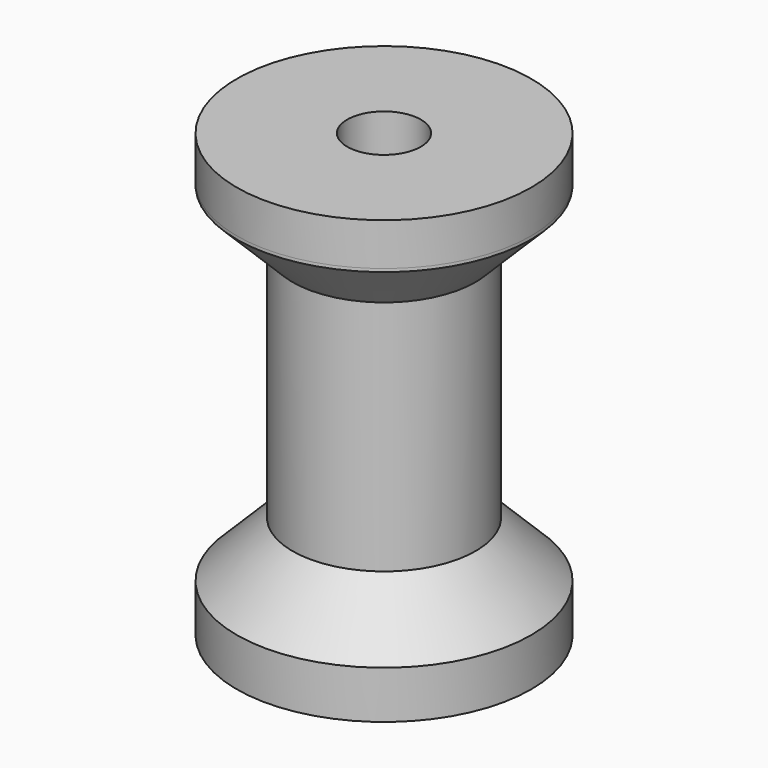
from build123d import *

# Parameters (mm, degrees)
F0_R         = 12.7
F1_DEPTH     = 38.1
F2_W         = 10.2602215484
F2_H         = 30.5833565071
F4_R         = 3.175
F5_DEPTH     = 50.8
F6_S5_R      = 12.7
F6_T6_DEPTH  = 20
F6_S11_R     = 12.7
F6_T12_DEPTH = 20


# Not quite as in the source:
# - a fillet or chamfer that OpenCascade refuses, or shapes differently, is made with other operations: its cross-section is extruded or revolved along the edge and cut away or added


with BuildPart() as f1:
    # F0 (on Top) → F1 (new body)
    with BuildSketch(Plane.XY):
        Circle(F0_R)
    extrude(amount=F1_DEPTH)

    # F2 (on Right) → F3 (revolve, cut)
    with BuildSketch(Plane.YZ):
        with Locations((-13.0225899629, 19.1392614506)):
            Rectangle(F2_W, F2_H)
    revolve(axis=Axis((0, 0, 18.941948656), (0, 0, -1)), mode=Mode.SUBTRACT)

    # F4 (on face) → F5 (cut)
    with BuildSketch(Plane(origin=(0, 0, 0), x_dir=(1, 0, 0), z_dir=(0, 0, -1))):
        Circle(F4_R)
    extrude(amount=-F5_DEPTH, mode=Mode.SUBTRACT)

    # F6: chamfer of 5.08 on 2 edges, made by hand


with BuildPart() as f6_tool2:
    # F6_s3 → F6_t4 (revolve)
    with BuildSketch(Plane.YZ):
        Polygon((-12.9724791887, 3.8475831971), (-7.8924791887, 8.9275831971), (-7.8924791887, 3.8475831971), align=None)
    revolve(axis=Axis((0, 0, 3.8475831971), (0, 0, -1)))

    # F6_s5 → F6_t6 (intersect, symmetric)
    with BuildSketch(Plane.XY.offset(6.4)):
        Circle(F6_S5_R)
    extrude(amount=F6_T6_DEPTH, both=True, mode=Mode.INTERSECT)


with BuildPart() as f1_1:
    add(f1.part)

    # F6_t1: union F6_tool2
    add(f6_tool2.part)


with BuildPart() as f6_tool8:
    # F6_s9 → F6_t10 (revolve)
    with BuildSketch(Plane.YZ):
        Polygon((-7.8924791887, 29.3509397042), (-12.9724791887, 34.4309397042), (-7.8924791887, 34.4309397042), align=None)
    revolve(axis=Axis((0, 0, 34.4309397042), (0, 0, -1)))

    # F6_s11 → F6_t12 (intersect, symmetric)
    with BuildSketch(Plane.XY.offset(31.9)):
        Circle(F6_S11_R)
    extrude(amount=F6_T12_DEPTH, both=True, mode=Mode.INTERSECT)


with BuildPart() as f1_2:
    add(f1_1.part)

    # F6_t7: union F6_tool8
    add(f6_tool8.part)


solid = f1_2.part
